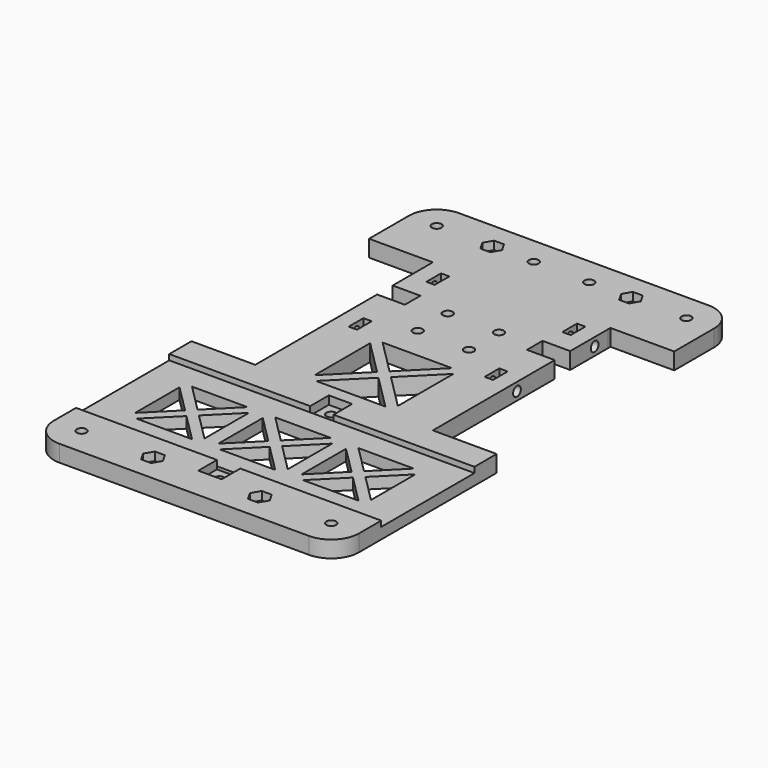
from build123d import *

# Parameters (mm, degrees)
F0_W      = 3
F0_H      = 6.6
F1_DEPTH  = 6
F2_R      = 1.75
F3_DEPTH  = 15
F4_R      = 1.75
F5_DEPTH  = 15
F6_R      = 1.75
F7_DEPTH  = 25
F9_DEPTH  = 3
F10_W     = 8.4
F10_H     = 8.4
F11_DEPTH = 3
F12_DEPTH = 2
F13_R     = 1.75
F14_DEPTH = 25
F15_R     = 1.75
F16_DEPTH = 25
F17_R     = 1.75
F18_DEPTH = 25
F20_DEPTH = 3
F21_R     = 1.75
F22_DEPTH = 25
F24_DEPTH = 3
F26_DEPTH = 25
F28_DEPTH = 25
F29_W     = 5.2
F29_H     = 16.75
F30_DEPTH = 2
F31_R     = 1.75
F32_DEPTH = 25
F33_R     = 1.75
F34_DEPTH = 3


# Not quite as in the source:
# - ends of sketch curves that miss each other by under 0.0002 mm in the source are joined
# - a feature names something its author has since deleted; it is built from what else it names


with BuildPart() as f1:
    # F0 (on Top) → F1 (new body)
    with BuildSketch(Plane.XY):
        with BuildLine():
            ThreePointArc((55, 95), (52.0710678119, 102.0710678119), (45, 105))
            Line((45, 105), (-45, 105))
            ThreePointArc((-45, 105), (-52.0710678119, 102.0710678119), (-55, 95))
            Line((-55, 95), (-55, 77))
            Line((-55, 77), (-32, 77))
            Line((-32, 77), (-32, 58.900007844))
            Line((-32, 58.900007844), (-21.9999993593, 58.900007844))
            Line((-21.9999993593, 58.900007844), (-21.9999993593, 51.900007844))
            Line((-21.9999993593, 51.900007844), (-31.9999993593, 51.900007844))
            Line((-31.9999993593, 51.900007844), (-32, -3))
            Line((-32, -3), (-55, -3))
            Line((-55, -3), (-55, -65))
            ThreePointArc((-55, -65), (-52.0710678119, -72.0710678119), (-45, -75))
            Line((-45, -75), (45, -75))
            ThreePointArc((45, -75), (52.0710678119, -72.0710678119), (55, -65))
            Line((55, -65), (55, -3))
            Line((55, -3), (32, -3))
            Line((32, -3), (32, 28.900007844))
            Line((32, 28.900007844), (32, 51.900007844))
            Line((32, 51.900007844), (21.9999993593, 51.900007844))
            Line((21.9999993593, 51.900007844), (21.9999993593, 58.900007844))
            Line((21.9999993593, 58.900007844), (31.9999993593, 58.900007844))
            Line((31.9999993593, 58.900007844), (32, 75.900007844))
            Line((32, 75.900007844), (32, 77))
            Line((32, 77), (55, 77))
            Line((55, 77), (55, 95))
        make_face()
        with Locations((-24.4999993593, 34.900007844)):
            Rectangle(F0_W, F0_H, mode=Mode.SUBTRACT)
        with Locations((-24.4999993593, 69.900007844)):
            Rectangle(F0_W, F0_H, mode=Mode.SUBTRACT)
        with Locations((24.4999993593, 34.900007844)):
            Rectangle(F0_W, F0_H, mode=Mode.SUBTRACT)
        with Locations((24.4999993593, 69.900007844)):
            Rectangle(F0_W, F0_H, mode=Mode.SUBTRACT)
    extrude(amount=F1_DEPTH)

    # F2 (on face) → F3 (cut)
    with BuildSketch(Plane.YZ.offset(32)):
        with Locations((34.9, 3)):
            Circle(F2_R)
        with Locations((69.9, 3)):
            Circle(F2_R)
    extrude(amount=-F3_DEPTH, mode=Mode.SUBTRACT)

    # F4 (on face) → F5 (cut)
    with BuildSketch(Plane(origin=(-32, 0, 0), x_dir=(0, -1, 0), z_dir=(-1, 0, 0))):
        with Locations((-69.9, 3)):
            Circle(F4_R)
        with Locations((-34.9, 3)):
            Circle(F4_R)
    extrude(amount=-F5_DEPTH, mode=Mode.SUBTRACT)

    # F6 (on face) → F7 (cut)
    with BuildSketch(Plane.XY.offset(6)):
        with Locations((-9.25, 55.25)):
            Circle(F6_R)
        with Locations((9.25, 55.25)):
            Circle(F6_R)
        with Locations((9.25, 41.75)):
            Circle(F6_R)
        with Locations((-9.25, 41.75)):
            Circle(F6_R)
    extrude(amount=-F7_DEPTH, mode=Mode.SUBTRACT)

    # F8 (on face) → F9 (cut)
    with BuildSketch(Plane(origin=(0, 0, 0), x_dir=(1, 0, 0), z_dir=(0, 0, -1))):
        Polygon((-7.4602141655, -38.65), (-11.0397858345, -38.65), (-12.829571669, -41.75), (-11.0397858345, -44.85), (-7.4602141655, -44.85), (-5.670428331, -41.75), align=None)
        Polygon((7.4602141655, -38.65), (5.670428331, -41.75), (7.4602141655, -44.85), (11.0397858345, -44.85), (12.829571669, -41.75), (11.0397858345, -38.65), align=None)
        Polygon((-7.5179491924, -52.25), (-10.9820508076, -52.25), (-12.7141016151, -55.25), (-10.9820508076, -58.25), (-7.5179491924, -58.25), (-5.7858983849, -55.25), align=None)
        Polygon((7.5179491924, -52.25), (5.7858983849, -55.25), (7.5179491924, -58.25), (10.9820508076, -58.25), (12.7141016151, -55.25), (10.9820508076, -52.25), align=None)
    extrude(amount=-F9_DEPTH, mode=Mode.SUBTRACT)

    # F10 (on face) → F11 (cut)
    with BuildSketch(Plane.XY.offset(6)):
        with Locations((0, -59.2)):
            Rectangle(F10_W, F10_H)
        with Locations((0, -8.8)):
            Rectangle(F10_W, F10_H)
    extrude(amount=-F11_DEPTH, mode=Mode.SUBTRACT)

    # F10 (on face) → F12 (cut)
    with BuildSketch(Plane.XY.offset(6)):
        Polygon((-4.2, -13), (-55, -13), (-55, -55), (-4.2, -55), (4.2, -55), (55, -55), (55, -13), (4.2, -13), align=None)
    extrude(amount=-F12_DEPTH, mode=Mode.SUBTRACT)

    # F13 (on face) → F14 (cut)
    with BuildSketch(Plane.XY.offset(3)):
        with Locations((0, -8.8)):
            Circle(F13_R)
        with Locations((0, -59.2)):
            Circle(F13_R)
    extrude(amount=-F14_DEPTH, mode=Mode.SUBTRACT)

    # F15 (on face) → F16 (cut)
    with BuildSketch(Plane.XY.offset(6)):
        with Locations((-45, 95)):
            Circle(F15_R)
        with Locations((45, 95)):
            Circle(F15_R)
        with Locations((45, -65)):
            Circle(F15_R)
        with Locations((-45, -65)):
            Circle(F15_R)
    extrude(amount=-F16_DEPTH, mode=Mode.SUBTRACT)

    # F17 (on face) → F18 (cut)
    with BuildSketch(Plane(origin=(0, 0, 0), x_dir=(1, 0, 0), z_dir=(0, 0, -1))):
        with Locations((-25, -95)):
            Circle(F17_R)
        with Locations((25, -95)):
            Circle(F17_R)
    extrude(amount=-F18_DEPTH, mode=Mode.SUBTRACT)

    # F19 (on face) → F20 (cut)
    with BuildSketch(Plane.XY.offset(6)):
        Polygon((-23.2102141655, 98.1), (-26.7897858345, 98.1), (-28.579571669, 95), (-26.7897858345, 91.9), (-23.2102141655, 91.9), (-21.420428331, 95), align=None)
        Polygon((23.2102141655, 91.9), (26.7897858345, 91.9), (28.579571669, 95), (26.7897858345, 98.1), (23.2102141655, 98.1), (21.420428331, 95), align=None)
    extrude(amount=-F20_DEPTH, mode=Mode.SUBTRACT)

    # F21 (on face) → F22 (cut)
    with BuildSketch(Plane(origin=(0, 0, 0), x_dir=(1, 0, 0), z_dir=(0, 0, -1))):
        with Locations((-10, -95)):
            Circle(F21_R)
        with Locations((10, -95)):
            Circle(F21_R)
    extrude(amount=-F22_DEPTH, mode=Mode.SUBTRACT)

    # F23 (on face) → F24 (cut)
    with BuildSketch(Plane(origin=(0, 0, 0), x_dir=(1, 0, 0), z_dir=(0, 0, -1))):
        Polygon((-8.2102141655, -91.9), (-11.7897858345, -91.9), (-13.579571669, -95), (-11.7897858345, -98.1), (-8.2102141655, -98.1), (-6.420428331, -95), align=None)
        Polygon((13.579571669, -95), (11.7897858345, -91.9), (8.2102141655, -91.9), (6.420428331, -95), (8.2102141655, -98.1), (11.7897858345, -98.1), align=None)
    extrude(amount=-F24_DEPTH, mode=Mode.SUBTRACT)

    # F25 (on face) → F26 (cut)
    with BuildSketch(Plane.XY.offset(6)):
        Polygon((0, 17.5), (12.5, 30), (-12.5, 30), align=None)
        Polygon((-15, 2.5), (-2.5, 15), (-15, 27.5), align=None)
        Polygon((12.5, 0), (0, 12.5), (-12.5, 0), align=None)
        Polygon((15, 2.5), (15, 27.5), (2.5, 15), align=None)
    extrude(amount=-F26_DEPTH, mode=Mode.SUBTRACT)

    # F27 (on face) → F28 (cut)
    with BuildSketch(Plane.XY.offset(4)):
        Polygon((-30, -36.5), (-40, -46.5), (-20, -46.5), align=None)
        Polygon((-40, -21.5), (-30, -31.5), (-20, -21.5), align=None)
        Polygon((-42.5, -24), (-42.5, -44), (-32.5, -34), align=None)
        Polygon((-17.5, -24), (-27.5, -34), (-17.5, -44), align=None)
        Polygon((10, -21.5), (-10, -21.5), (0, -31.5), align=None)
        Polygon((12.5, -24), (2.5, -34), (12.5, -44), align=None)
        Polygon((-12.5, -44), (-2.5, -34), (-12.5, -24), align=None)
        Polygon((10, -46.5), (0, -36.5), (-10, -46.5), align=None)
        Polygon((40, -21.5), (20, -21.5), (30, -31.5), align=None)
        Polygon((42.5, -24), (32.5, -34), (42.5, -44), align=None)
        Polygon((17.5, -44), (27.5, -34), (17.5, -24), align=None)
        Polygon((40, -46.5), (30, -36.5), (20, -46.5), align=None)
    extrude(amount=-F28_DEPTH, mode=Mode.SUBTRACT)

    # F29 (on face) → F30 (cut)
    with BuildSketch(Plane(origin=(0, 0, 0), x_dir=(1, 0, 0), z_dir=(0, 0, -1))):
        with Locations((-25, -96.625)):
            Rectangle(F29_W, F29_H)
        with Locations((25, -96.625)):
            Rectangle(F29_W, F29_H)
    extrude(amount=-F30_DEPTH, mode=Mode.SUBTRACT)

    # F31 (on face) → F32 (cut)
    with BuildSketch(Plane(origin=(0, 0, 0), x_dir=(1, 0, 0), z_dir=(0, 0, -1))):
        with Locations((-19.25, 65)):
            Circle(F31_R)
        with Locations((19.25, 65)):
            Circle(F31_R)
    extrude(amount=-F32_DEPTH, mode=Mode.SUBTRACT)

    # F33 (on face) → F34 (cut)
    with BuildSketch(Plane.XY.offset(6)):
        Polygon((-17.4602141655, -61.9), (-21.0397858345, -61.9), (-22.829571669, -65), (-21.0397858345, -68.1), (-17.4602141655, -68.1), (-15.670428331, -65), align=None)
        with Locations((-19.25, -65)):
            Circle(F33_R, mode=Mode.SUBTRACT)
        Polygon((17.4602141655, -61.9), (15.670428331, -65), (17.4602141655, -68.1), (21.0397858345, -68.1), (22.829571669, -65), (21.0397858345, -61.9), align=None)
        with Locations((19.25, -65)):
            Circle(F33_R, mode=Mode.SUBTRACT)
    extrude(amount=-F34_DEPTH, mode=Mode.SUBTRACT)


solid = f1.part
